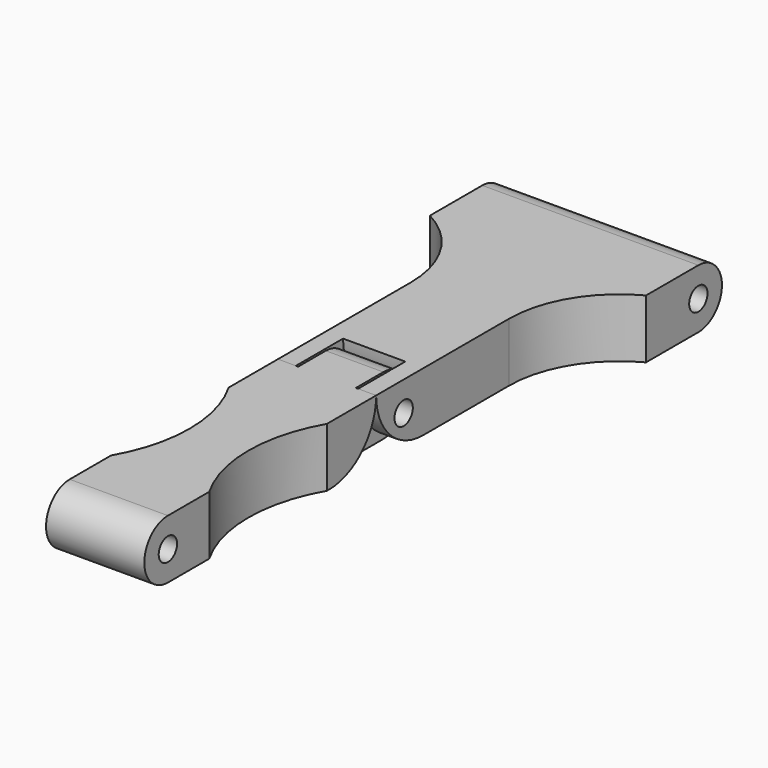
from build123d import *

# Parameters (mm, degrees)
F1_DEPTH  = 7.5
F3_DEPTH  = 4.4
F4_R      = 22.5
F5_DEPTH  = 25
F9_DEPTH  = 16.5
F11_DEPTH = 25
F13_W     = 9.5
F13_H     = 11.25
F14_DEPTH = 25
F16_R     = 8.99999
F17_R     = 1.75
F18_DEPTH = 40


# Not quite as in the source:
# - a fillet or chamfer is up to 0.001 mm smaller than in the source, because OpenCascade refuses the exact size


with BuildPart() as f1:
    # F0 (on Right) → F1 (new body, symmetric)
    with BuildSketch(Plane.YZ):
        with BuildLine():
            ThreePointArc((-22.5, 9), (-27, 4.5), (-22.5, 0))
            Line((-22.5, 0), (8.25, 0))
            ThreePointArc((8.25, 0), (14.6139610307, 2.6360389693), (17.25, 9))
            Line((17.25, 9), (-22.5, 9))
        make_face()
    extrude(amount=F1_DEPTH, both=True)

    # F2 (on Right) → F3 (join, symmetric)
    with BuildSketch(Plane.YZ):
        with BuildLine():
            Line((22.5, 9), (0, 9))
            Line((0, 9), (0, 0))
            Line((0, 0), (22.5, 0))
            ThreePointArc((22.5, 0), (27, 4.5), (22.5, 9))
        make_face()
    extrude(amount=F3_DEPTH, both=True)


with BuildPart() as f5:
    # F4 (on Top) → F5 (new body)
    with BuildSketch(Plane.XY):
        with Locations((-27, -3.375)):
            Circle(F4_R)
    extrude(amount=F5_DEPTH)


with BuildPart() as f6_1:
    # F6: instance of F5
    add(f5.part.mirror(Plane.YZ))


with BuildPart() as f1_1:
    add(f1.part)

    # F7: cut F6_1, F5
    add(f6_1.part, mode=Mode.SUBTRACT)
    add(f5.part, mode=Mode.SUBTRACT)


with BuildPart() as f9:
    # F8 (on Right) → F9 (new body, symmetric)
    with BuildSketch(Plane.YZ):
        with BuildLine():
            Line((67.5, 9), (17.25, 9))
            ThreePointArc((17.25, 9), (19.8860389693, 2.6360389693), (26.25, 0))
            Line((26.25, 0), (67.5, 0))
            ThreePointArc((67.5, 0), (72, 4.5), (67.5, 9))
        make_face()
    extrude(amount=F9_DEPTH, both=True)


with BuildPart() as f11:
    # F10 (on Top) → F11 (new body)
    with BuildSketch(Plane.XY):
        with BuildLine():
            Line((7.5, 42.6077849247), (7.5, 16.5))
            Line((7.5, 16.5), (18.75, 16.5))
            Line((18.75, 16.5), (18.75, 58.5))
            ThreePointArc((18.75, 58.5), (10.5971366618, 52.343351164), (7.5, 42.6077849247))
        make_face()
    extrude(amount=F11_DEPTH)


with BuildPart() as f12_1:
    # F12: instance of F11
    add(f11.part.mirror(Plane.YZ))


with BuildPart() as f14:
    # F13 (on Top) → F14 (new body)
    with BuildSketch(Plane.XY):
        with Locations((0, 20.625)):
            Rectangle(F13_W, F13_H)
    extrude(amount=F14_DEPTH)


with BuildPart() as f9_1:
    add(f9.part)

    # F15: cut F12_1, F11, F14
    add(f12_1.part, mode=Mode.SUBTRACT)
    add(f11.part, mode=Mode.SUBTRACT)
    add(f14.part, mode=Mode.SUBTRACT)

    # F16 (radius 9 in the source; OpenCascade refuses exactly that, so slightly less here)
    f16_edges = [f9_1.edges().sort_by_distance(p)[0] for p in [
        (6.125, 26.25, 0),
        (0, 26.25, 0),
        (-6.125, 26.25, 0),
    ]]
    fillet(f16_edges, radius=F16_R)


with BuildPart() as f18:
    # F17 (on face) → F18 (new body, symmetric)
    with BuildSketch(Plane.YZ.offset(7.5)):
        with Locations((-22.5, 4.5)):
            Circle(F17_R)
    extrude(amount=F18_DEPTH, both=True)


with BuildPart() as f18b:
    # F17 (on face) → F18, piece 2 (new body, symmetric)
    with BuildSketch(Plane.YZ.offset(7.5)):
        with Locations((22.5, 4.5)):
            Circle(F17_R)
    extrude(amount=F18_DEPTH, both=True)


with BuildPart() as f18c:
    # F17 (on face) → F18, piece 3 (new body, symmetric)
    with BuildSketch(Plane.YZ.offset(7.5)):
        with Locations((67.5, 4.5)):
            Circle(F17_R)
    extrude(amount=F18_DEPTH, both=True)


with BuildPart() as f1_2:
    add(f1_1.part)

    # F19: cut F18b, F18, F18c
    add(f18b.part, mode=Mode.SUBTRACT)
    add(f18.part, mode=Mode.SUBTRACT)
    add(f18c.part, mode=Mode.SUBTRACT)


with BuildPart() as f9_2:
    add(f9_1.part)

    # F19: cut F18b, F18, F18c
    add(f18b.part, mode=Mode.SUBTRACT)
    add(f18.part, mode=Mode.SUBTRACT)
    add(f18c.part, mode=Mode.SUBTRACT)


solid = Compound([f1_2.part, f9_2.part])
